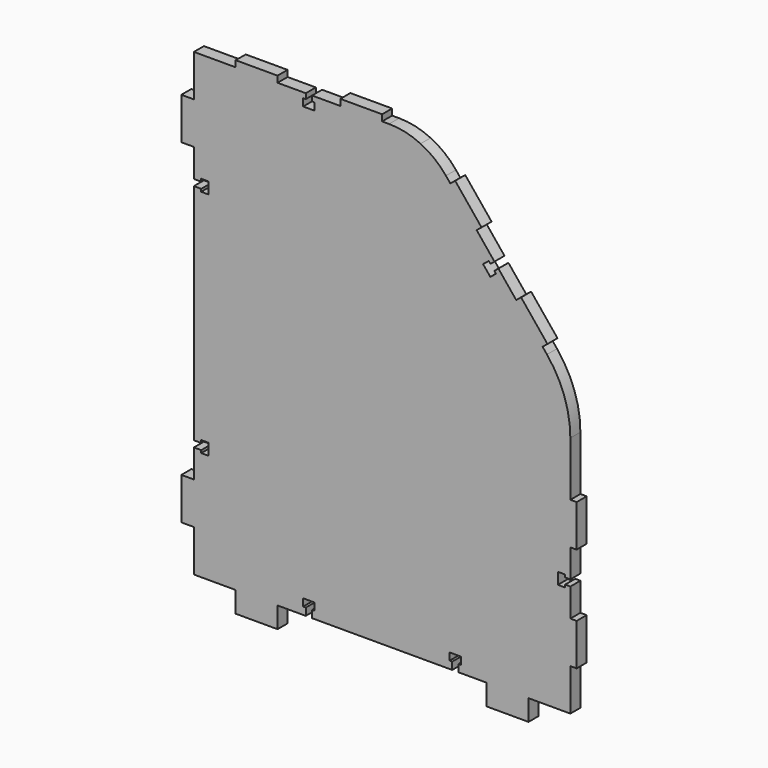
from build123d import *

# Parameters (mm, degrees)
F1_DEPTH = 6


# Not quite as in the source:
# - a feature names something its author has since deleted; it is built from what else it names


with BuildPart() as f1:
    # F0 (on Front) → F1 (new body)
    with BuildSketch(Plane.XZ):
        with BuildLine():
            Line((20, 220), (0, 220))
            Line((0, 220), (0, 200))
            Line((0, 200), (-6, 200))
            Line((-6, 200), (-6, 180))
            Line((-6, 180), (0, 180))
            Line((0, 180), (0, 166.5))
            Line((0, 166.5), (3.5, 166.5))
            Line((3.5, 166.5), (3.5, 167.75))
            Line((3.5, 167.75), (7, 167.75))
            Line((7, 167.75), (7, 162.25))
            Line((7, 162.25), (3.5, 162.25))
            Line((3.5, 162.25), (3.5, 163.5))
            Line((3.5, 163.5), (0, 163.5))
            Line((0, 163.5), (0, 110))
            Line((0, 110), (0, 56.5))
            Line((0, 56.5), (3.5, 56.5))
            Line((3.5, 56.5), (3.5, 57.75))
            Line((3.5, 57.75), (7, 57.75))
            Line((7, 57.75), (7, 52.25))
            Line((7, 52.25), (3.5, 52.25))
            Line((3.5, 52.25), (3.5, 53.5))
            Line((3.5, 53.5), (0, 53.5))
            Line((0, 53.5), (0, 40))
            Line((0, 40), (-6, 40))
            Line((-6, 40), (-6, 20))
            Line((-6, 20), (0, 20))
            Line((0, 20), (0, 0))
            Line((0, 0), (20, 0))
            Line((20, 0), (20, -10))
            Line((20, -10), (40, -10))
            Line((40, -10), (40, 0))
            Line((40, 0), (53.5, 0))
            Line((53.5, 0), (53.5, 3.5))
            Line((53.5, 3.5), (52.25, 3.5))
            Line((52.25, 3.5), (52.25, 7))
            Line((52.25, 7), (57.75, 7))
            Line((57.75, 7), (57.75, 3.5))
            Line((57.75, 3.5), (56.5, 3.5))
            Line((56.5, 3.5), (56.5, 0))
            Line((56.5, 0), (90, 0))
            Line((90, 0), (123.5, 0))
            Line((123.5, 0), (123.5, 3.5))
            Line((123.5, 3.5), (122.25, 3.5))
            Line((122.25, 3.5), (122.25, 7))
            Line((122.25, 7), (127.75, 7))
            Line((127.75, 7), (127.75, 3.5))
            Line((127.75, 3.5), (126.5, 3.5))
            Line((126.5, 3.5), (126.5, 0))
            Line((126.5, 0), (140, 0))
            Line((140, 0), (140, -10))
            Line((140, -10), (160, -10))
            Line((160, -10), (160, 0))
            Line((160, 0), (180, 0))
            Line((180, 0), (180, 20))
            Line((180, 20), (183, 20))
            Line((183, 20), (183, 40))
            Line((183, 40), (180, 40))
            Line((180, 40), (180, 53.5))
            Line((180, 53.5), (177.5, 53.5))
            Line((177.5, 53.5), (177.5, 52.25))
            Line((177.5, 52.25), (174, 52.25))
            Line((174, 52.25), (174, 57.75))
            Line((174, 57.75), (177.5, 57.75))
            Line((177.5, 57.75), (177.5, 56.5))
            Line((177.5, 56.5), (180, 56.5))
            Line((180, 56.5), (180, 70))
            Line((180, 70), (183, 70))
            Line((183, 70), (183, 90))
            Line((183, 90), (180, 90))
            Line((180, 90), (180, 110))
            Line((180, 110), (180, 116.0255279073))
            ThreePointArc((180, 116.0255279073), (177.1222639523, 132.7435493216), (168.8203103996, 147.5371686211))
            Line((168.8203103996, 147.5371686211), (166.7209532849, 150.1234412807))
            Line((166.7209532849, 150.1234412807), (169.0501719088, 152.0141397235))
            Line((169.0501719088, 152.0141397235), (156.4455156233, 167.5422638833))
            Line((156.4455156233, 167.5422638833), (154.1162969993, 165.6515654405))
            Line((154.1162969993, 165.6515654405), (145.6081540066, 176.1330492484))
            Line((145.6081540066, 176.1330492484), (143.6671384866, 174.5574672127))
            Line((143.6671384866, 174.5574672127), (144.4549295045, 173.5869594527))
            Line((144.4549295045, 173.5869594527), (141.7375077765, 171.3811446028))
            Line((141.7375077765, 171.3811446028), (138.271227298, 175.6513787467))
            Line((138.271227298, 175.6513787467), (140.988649026, 177.8571935967))
            Line((140.988649026, 177.8571935967), (141.7764400438, 176.8866858367))
            Line((141.7764400438, 176.8866858367), (143.7174555638, 178.4622678724))
            Line((143.7174555638, 178.4622678724), (135.2093125711, 188.9437516803))
            Line((135.2093125711, 188.9437516803), (137.538531195, 190.8344501231))
            Line((137.538531195, 190.8344501231), (124.9338749095, 206.362574283))
            Line((124.9338749095, 206.362574283), (122.6046562855, 204.4718758401))
            Line((122.6046562855, 204.4718758401), (120.5052991708, 207.0581484997))
            ThreePointArc((120.5052991708, 207.0581484997), (114.9751472562, 212.5051710496), (108.3804141438, 216.5993290869))
            ThreePointArc((108.3804141438, 216.5993290869), (101.0454672184, 219.1392480735), (93.331081891, 220))
            Line((93.331081891, 220), (90, 220))
            Line((90, 220), (90, 223))
            Line((90, 223), (70, 223))
            Line((70, 223), (70, 220))
            Line((70, 220), (56.5, 220))
            Line((56.5, 220), (56.5, 217.5))
            Line((56.5, 217.5), (57.75, 217.5))
            Line((57.75, 217.5), (57.75, 214))
            Line((57.75, 214), (52.25, 214))
            Line((52.25, 214), (52.25, 217.5))
            Line((52.25, 217.5), (53.5, 217.5))
            Line((53.5, 217.5), (53.5, 220))
            Line((53.5, 220), (40, 220))
            Line((40, 220), (40, 223))
            Line((40, 223), (20, 223))
            Line((20, 223), (20, 220))
        make_face()
    extrude(amount=F1_DEPTH)


solid = f1.part
